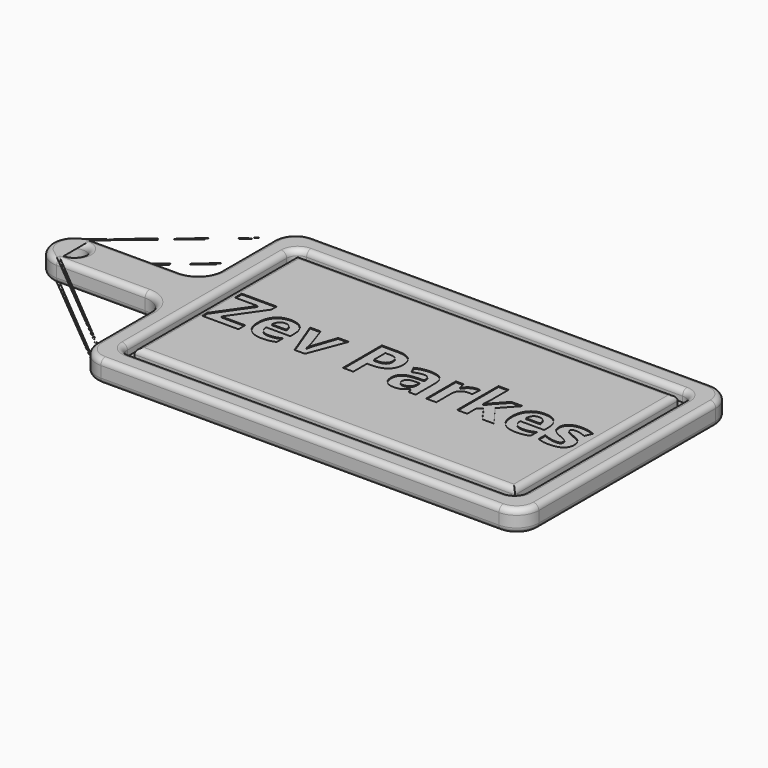
from build123d import *

# Parameters (mm, degrees)
F0_W          = 76.2
F0_H          = 25.4
F1_DEPTH      = 12.7
F2_R          = 6.35
F3_DEPTH      = 25.4
F5_DEPTH      = 6.35
F6_R          = 6.35
F7_R          = 12.7
F8_R          = 12.69999
F9_R          = 3.17499
F10_TEXT_SIZE = 39.1343808563
F11_DEPTH     = 0.508


# Not quite as in the source:
# - a fillet or chamfer is up to 0.001 mm smaller than in the source, because OpenCascade refuses the exact size
# - Text() gives the source's letters only with a copy of the font that has no kerning and outlines rounded to 1/6400 em; it was checked with that copy


with BuildPart() as f1:
    # F0 (on Top) → F1 (new body)
    with BuildSketch(Plane.XY):
        Polygon((0, 63.5), (0, 0), (254, 0), (254, 152.4), (0, 152.4), (0, 88.9), align=None)
        with Locations((-38.1, 76.2)):
            Rectangle(F0_W, F0_H)
    extrude(amount=F1_DEPTH)

    # F2 (on face) → F3 (cut)
    with BuildSketch(Plane.XY.offset(12.7)):
        with Locations((-63.5, 76.2)):
            Circle(F2_R)
    extrude(amount=-F3_DEPTH, mode=Mode.SUBTRACT)

    # F4 (on face) → F5 (cut)
    with BuildSketch(Plane.XY.offset(12.7)):
        Polygon((12.7, 63.5), (12.7, 12.7), (241.3, 12.7), (241.3, 139.7), (12.7, 139.7), (12.7, 88.9), align=None)
        Polygon((17.78, 63.5), (17.78, 88.9), (17.78, 134.62), (236.22, 134.62), (236.22, 17.78), (17.78, 17.78), align=None, mode=Mode.SUBTRACT)
    extrude(amount=-F5_DEPTH, mode=Mode.SUBTRACT)

    # F6
    f6_edges = [f1.edges().sort_by_distance(p)[0] for p in [
        (12.7, 139.7, 9.525),
        (12.7, 12.7, 9.525),
        (241.3, 139.7, 9.525),
        (241.3, 12.7, 9.525),
    ]]
    fillet(f6_edges, radius=F6_R)

    # F7
    f7_edges = [f1.edges().sort_by_distance(p)[0] for p in [
        (0, 152.4, 6.35),
        (254, 152.4, 6.35),
        (254, 0, 6.35),
        (0, 0, 6.35),
    ]]
    fillet(f7_edges, radius=F7_R)

    # F8 (radius 12.7 in the source; OpenCascade refuses exactly that, so slightly less here)
    f8_edges = [f1.edges().sort_by_distance(p)[0] for p in [
        (-76.2, 63.5, 6.35),
        (-76.2, 88.9, 6.35),
        (0, 63.5, 6.35),
        (0, 88.9, 6.35),
    ]]
    fillet(f8_edges, radius=F8_R)

    # F9 (radius 3.175 in the source; OpenCascade refuses exactly that, so slightly less here)
    f9_edges = [f1.edges().sort_by_distance(p)[0] for p in [
        (127, 134.62, 12.7),
        (236.22, 76.2, 12.7),
        (127, 17.78, 12.7),
        (17.78, 76.2, 12.7),
        (0, 31.750005, 12.7),
        (-3.719741, 59.780259, 12.7),
        (3.719744, 3.719744, 12.7),
        (-38.1, 63.5, 12.7),
        (127, 0, 12.7),
        (-72.480259, 67.219741, 12.7),
        (250.280256, 3.719744, 12.7),
        (-76.2, 76.2, 12.7),
        (254, 76.2, 12.7),
        (-72.480259, 85.180259, 12.7),
        (250.280256, 148.680256, 12.7),
        (-38.1, 88.9, 12.7),
        (127, 152.4, 12.7),
        (-3.719741, 92.619741, 12.7),
        (3.719744, 148.680256, 12.7),
        (0, 120.649995, 12.7),
        (127, 12.7, 12.7),
        (14.559872, 14.559872, 12.7),
        (239.440128, 14.559872, 12.7),
        (12.7, 76.2, 12.7),
        (241.3, 76.2, 12.7),
        (14.559872, 137.840128, 12.7),
        (239.440128, 137.840128, 12.7),
        (127, 139.7, 12.7),
        (-69.85, 76.2, 12.7),
        (0, 31.750005, 0),
        (-3.719741, 59.780259, 0),
        (3.719744, 3.719744, 0),
        (-38.1, 63.5, 0),
        (127, 0, 0),
        (-72.480259, 67.219741, 0),
        (250.280256, 3.719744, 0),
        (-76.2, 76.2, 0),
        (254, 76.2, 0),
        (-72.480259, 85.180259, 0),
        (250.280256, 148.680256, 0),
        (-38.1, 88.9, 0),
        (127, 152.4, 0),
        (-3.719741, 92.619741, 0),
        (3.719744, 148.680256, 0),
        (0, 120.649995, 0),
        (-69.85, 76.2, 0),
    ]]
    fillet(f9_edges, radius=F9_R)

    # F10 (on face) → F11 (cut)
    with BuildSketch(Plane.XY.offset(12.7)):
        with Locations((20.955, 61.2411848372)):
            Text('Zev Parkes', F10_TEXT_SIZE, font='Open Sans', font_style=FontStyle.BOLD, text_align=(TextAlign.LEFT, TextAlign.BOTTOM))
    extrude(amount=-F11_DEPTH, mode=Mode.SUBTRACT)


solid = f1.part
